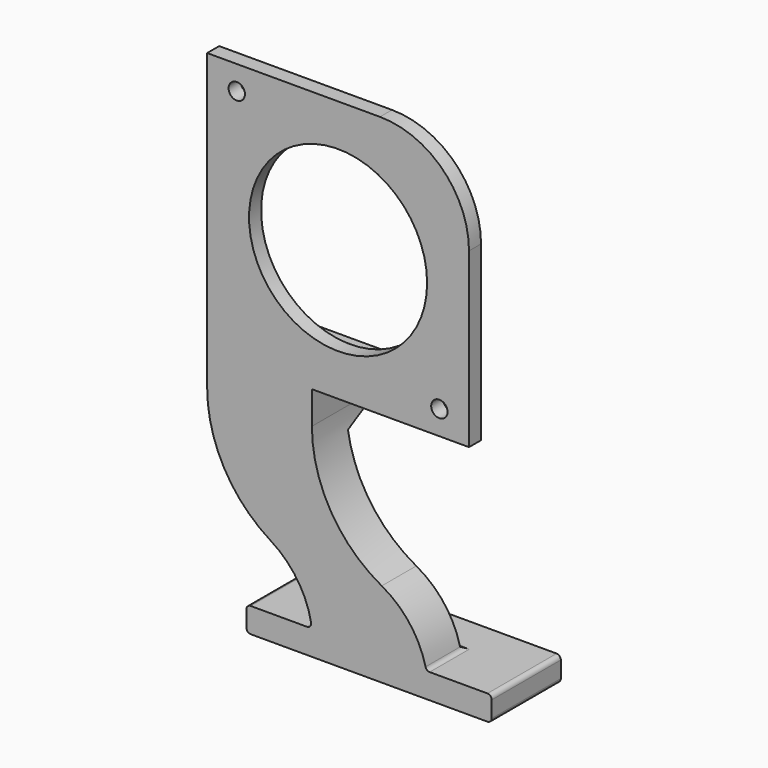
from build123d import *

# Parameters (mm, degrees)
F0_R        = 1.5875
F0_R_2      = 17.272
F1_DEPTH    = 2.921
F3_DEPTH    = 20.32
F5_DEPTH    = 16.764
F7_DEPTH    = 55.2085729102
F8_T        = 1.5875
F8_T3_DEPTH = 6.096
F8_T5_DEPTH = 23.495
F8_T7_DEPTH = 25.3893680424
F8_T9_DEPTH = 27.0060511967


# Not quite as in the source:
# - a shell that OpenCascade refuses in one call is made with other operations: the cavity is built on its own and cut out


with BuildPart() as f1:
    # F0 (on Front) → F1 (new body)
    with BuildSketch(Plane.XZ):
        with BuildLine():
            Line((-808.7745012016, 183.0527484417), (-842.3025012016, 183.0527484417))
            Line((-842.3025012016, 183.0527484417), (-842.3025012016, 132.2527484417))
            Line((-842.3025012016, 132.2527484417), (-791.5025012016, 132.2527484417))
            Line((-791.5025012016, 132.2527484417), (-791.5025012016, 165.7807484417))
            ThreePointArc((-791.5025012016, 165.7807484417), (-796.561352877, 177.9938967664), (-808.7745012016, 183.0527484417))
        make_face()
        with Locations((-797.2470434503, 136.9116393686)):
            Circle(F0_R, mode=Mode.SUBTRACT)
        with Locations((-816.9025012016, 157.6527484417)):
            Circle(F0_R_2, mode=Mode.SUBTRACT)
        with Locations((-836.557958953, 178.3938575148)):
            Circle(F0_R, mode=Mode.SUBTRACT)
    extrude(amount=F1_DEPTH)

    # F2 (on face) → F3 (join)
    with BuildSketch(Plane(origin=(-842.3025012016, 0, 0), x_dir=(0, -1, 0), z_dir=(-1, 0, 0))):
        Polygon((2.921, 125.9027484417), (2.921, 132.2527484417), (0, 132.2527484417), (-13.843, 132.2527484417), (-13.843, 125.9027484417), align=None)
    extrude(amount=-F3_DEPTH)

    # F4 (on face) → F5 (join, through all)
    with BuildSketch(Plane.XZ.offset(2.921)):
        with BuildLine():
            Line((-821.9825012016, 125.9027484417), (-842.3025012016, 125.9027484417))
            ThreePointArc((-842.3025012016, 125.9027484417), (-839.0194061041, 113.2468388218), (-829.9981379746, 103.782828939))
            ThreePointArc((-829.9981379746, 103.782828939), (-824.8710634373, 98.8883942721), (-822.1415983833, 92.3468039044))
            ThreePointArc((-822.1415983833, 92.3468039044), (-822.3177482435, 91.6604679901), (-822.9588808932, 91.3587484417))
            Line((-822.9588808932, 91.3587484417), (-833.8504607139, 91.3587484417))
            ThreePointArc((-833.8504607139, 91.3587484417), (-834.438802185, 91.115049425), (-834.6825012016, 90.5267079539))
            Line((-834.6825012016, 90.5267079539), (-834.6825012016, 87.3647889295))
            ThreePointArc((-834.6825012016, 87.3647889295), (-834.438802185, 86.7764474583), (-833.8504607139, 86.5327484417))
            Line((-833.8504607139, 86.5327484417), (-787.9259687792, 86.5327484417))
            ThreePointArc((-787.9259687792, 86.5327484417), (-787.337627308, 86.7764474583), (-787.0939282914, 87.3647889295))
            Line((-787.0939282914, 87.3647889295), (-787.0939282914, 90.5267079539))
            ThreePointArc((-787.0939282914, 90.5267079539), (-787.337627308, 91.115049425), (-787.9259687792, 91.3587484417))
            Line((-787.9259687792, 91.3587484417), (-799.1278296965, 91.3587484417))
            ThreePointArc((-799.1278296965, 91.3587484417), (-799.6417555246, 91.5364406915), (-799.9361712736, 91.9936208083))
            ThreePointArc((-799.9361712736, 91.9936208083), (-803.0180469013, 98.4212453171), (-808.4330915744, 103.0569335505))
            ThreePointArc((-808.4330915744, 103.0569335505), (-818.3403970657, 112.6219563033), (-821.9825012016, 125.9027484417))
        make_face()
    extrude(amount=-F5_DEPTH)

    # F6 (on face) → F7 (cut, through all)
    with BuildSketch(Plane.YZ.offset(-787.0939282914)):
        Polygon((13.843, 91.3587484417), (13.843, 125.9027484417), (5.461, 122.0099536731), (5.461, 91.9936208083), (6.6532706411, 91.3587484417), align=None)
    extrude(amount=-F7_DEPTH, mode=Mode.SUBTRACT)

    # F8: shell of thickness 1.5875, made by hand


with BuildPart() as f8_core1:
    # F8_t2: copy of F1
    add(f1.part)

    # the walls: a layer under each face that stays
    f8_faces = [f8_core1.faces().sort_by_distance(p)[0] for p in [
        (-825.5385012016, -1.4605, 183.0527484417),
        (-814.6982147465, -2.921, 134.7927484417),
        (-838.145458953, -1.4605, 178.3938575148),
        (-834.1745012016, -1.4605, 157.6527484417),
        (-798.8345434503, -1.4605, 136.9116393686),
        (-791.5025012016, -1.4605, 149.0167484417),
        (-806.7425012016, -1.4605, 132.2527484417),
        (-821.9825012016, 5.461, 129.0777484417),
        (-832.1425012016, 13.843, 129.0777484417),
        (-831.9961644541, 9.652, 123.9563510574),
        (-820.9729994901, 5.461, 107.0017872407),
        (-811.0433552949, 6.0571353205, 91.676184625),
        (-812.2898246487, -0.127, 105.6357879061),
        (-803.0180469013, 1.27, 98.4212453171),
        (-799.6417555246, 1.8661353205, 91.5364406915),
        (-787.0939282914, 5.461, 88.9457484417),
        (-810.8882147465, 5.461, 86.5327484417),
        (-834.6825012016, 5.461, 88.9457484417),
        (-795.5800507683, 11.049, 91.3587484417),
        (-822.3177482435, 1.8661353205, 91.6604679901),
        (-824.8710634373, 1.27, 98.8883942721),
        (-841.9306657608, -0.127, 121.5183203365),
        (-833.835834535, 0, 140.7194151084),
        (-842.3025012016, -0.127, 173.5277484417),
        (-796.561352877, -1.4605, 177.9938967664),
    ]]
    thicken(f8_faces, amount=-F8_T, mode=Mode.SUBTRACT)

    # F8_s4 → F8_t3 (cut)
    with BuildSketch(Plane.XZ.offset(-1.5875)):
        Polygon((-821.9666262016, 132.2368734417), (-821.9825012016, 133.8402484417), (-823.5700012016, 133.8402484417), (-823.5700012016, 132.2527484417), align=None)
    extrude(amount=F8_T3_DEPTH, mode=Mode.SUBTRACT)

    # F8_s6 → F8_t5 (cut)
    with BuildSketch(Plane.YZ.offset(-843.5973277066)):
        Polygon((5.4835617697, 121.9955556616), (4.7923230267, 123.4497548244), (3.8735, 123.0230321483), (3.8735, 122.0099536731), align=None)
    extrude(amount=F8_T5_DEPTH, mode=Mode.SUBTRACT)

    # F8_s8 → F8_t7 (cut)
    with BuildSketch(Plane.YZ.offset(-823.7380393161)):
        Polygon((5.4843363881, 92.0076330641), (3.8735, 91.9936208083), (3.8735, 91.0404117704), (4.7148611881, 90.5923952293), align=None)
    extrude(amount=F8_T7_DEPTH, mode=Mode.SUBTRACT)

    # F8_s10 → F8_t9 (cut)
    with BuildSketch(Plane.YZ.offset(-824.5463808932)):
        Polygon((6.6607320292, 91.3886356975), (5.9071318292, 89.9575228626), (6.2569494224, 89.7712484417), (6.6532706411, 89.7712484417), align=None)
    extrude(amount=F8_T9_DEPTH, mode=Mode.SUBTRACT)


with BuildPart() as f1_1:
    add(f1.part)

    # what is left inside the walls is the cavity
    f8_cavity = [f8_core1.part.solids().sort_by_distance(p)[0] for p in [
        (-814.698215, -1.317625, 102.831082),
    ]]
    add(f8_cavity, mode=Mode.SUBTRACT)


solid = f1_1.part
